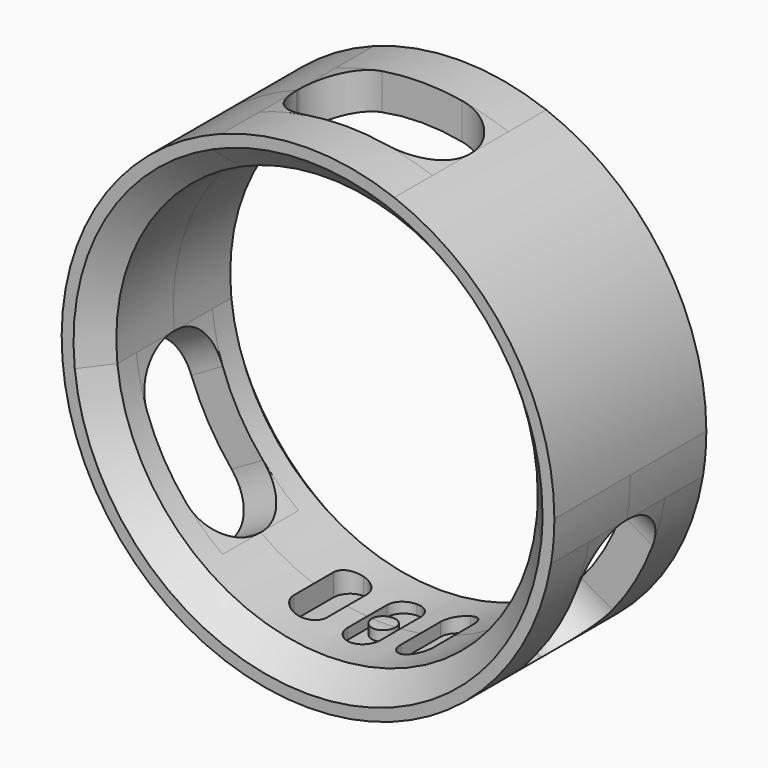
from build123d import *

# Parameters (mm, degrees)
F1_DEPTH      = 4
F1_DEPTH_BACK = 4
F2_SIZE       = 1
F4_DEPTH      = 2
F4_DEPTH_BACK = 2
F5_T4_DEPTH   = 11.3208024162
F5_S5_R       = 8.875
F5_T6_DEPTH   = 8
F5_S7_R       = 10.375
F5_T8_DEPTH   = 8
F5_T12_DEPTH  = 11.3208024162
F5_S13_R      = 10.375
F5_T14_DEPTH  = 8
F5_S15_R      = 8.875
F5_T16_DEPTH  = 8
F5_T20_DEPTH  = 11.3208024162
F5_S21_R      = 8.875
F5_T22_DEPTH  = 8
F5_S23_R      = 10.375
F5_T24_DEPTH  = 8
F5_T28_DEPTH  = 11.3208024162
F5_S29_R      = 8.875
F5_T30_DEPTH  = 8
F5_S31_R      = 10.375
F5_T32_DEPTH  = 8
F5_T36_DEPTH  = 11.3208024162
F5_S37_R      = 8.875
F5_T38_DEPTH  = 8
F5_S39_R      = 10.375
F5_T40_DEPTH  = 8
F5_T44_DEPTH  = 11.3208024162
F5_S45_R      = 8.875
F5_T46_DEPTH  = 8
F5_S47_R      = 10.375
F5_T48_DEPTH  = 8
F5_T52_DEPTH  = 11.3208024162
F5_S53_R      = 8.875
F5_T54_DEPTH  = 8
F5_S55_R      = 10.375
F5_T56_DEPTH  = 8
F5_T60_DEPTH  = 11.3208024162
F5_S61_R      = 8.875
F5_T62_DEPTH  = 8
F5_S63_R      = 10.375
F5_T64_DEPTH  = 8
F5_T68_DEPTH  = 11.3208024162
F5_S69_R      = 8.875
F5_T70_DEPTH  = 7
F5_S71_R      = 10.375
F5_T72_DEPTH  = 7
F5_T76_DEPTH  = 11.3208024162
F5_S77_R      = 8.875
F5_T78_DEPTH  = 7
F5_S79_R      = 10.375
F5_T80_DEPTH  = 7
F5_T84_DEPTH  = 11.3208024162
F5_S85_R      = 8.875
F5_T86_DEPTH  = 7
F5_S87_R      = 10.375
F5_T88_DEPTH  = 7
F5_T92_DEPTH  = 11.3208024162
F5_S93_R      = 8.875
F5_T94_DEPTH  = 7
F5_S95_R      = 10.375
F5_T96_DEPTH  = 7
F6_R          = 0.5
F7_DEPTH      = 9.3


# Not quite as in the source:
# - a fillet or chamfer that OpenCascade refuses, or shapes differently, is made with other operations: its cross-section is extruded or revolved along the edge and cut away or added


with BuildPart() as f1:
    # F0 (on Front) → F1 (new body, two sides)
    with BuildSketch(Plane.XZ) as f1_sk:
        with BuildLine():
            ThreePointArc((-3.6332620451, 8.0972237163), (0, 8.875), (3.6332620451, 8.0972237163))
            Line((3.6332620451, 8.0972237163), (3.6332620451, 9.7180261325))
            ThreePointArc((3.6332620451, 9.7180261325), (0, 10.375), (-3.6332620451, 9.7180261325))
            Line((-3.6332620451, 9.7180261325), (-3.6332620451, 8.0972237163))
        make_face()
        with BuildLine():
            ThreePointArc((-8.829032461, -0.9021146285), (-7.6859754586, 4.4375), (-3.6332620451, 8.0972237163))
            Line((-3.6332620451, 8.0972237163), (-3.6332620451, 9.7180261325))
            ThreePointArc((-3.6332620451, 9.7180261325), (-8.9850135643, 5.1875), (-10.2326885279, -1.7125158366))
            Line((-10.2326885279, -1.7125158366), (-8.829032461, -0.9021146285))
        make_face()
        with BuildLine():
            ThreePointArc((-5.1957704159, -7.1951090878), (-7.6859754586, -4.4375), (-8.829032461, -0.9021146285))
            Line((-8.829032461, -0.9021146285), (-10.2326885279, -1.7125158366))
            ThreePointArc((-10.2326885279, -1.7125158366), (-8.9850135643, -5.1875), (-6.5994264829, -8.0055102959))
            Line((-6.5994264829, -8.0055102959), (-5.1957704159, -7.1951090878))
        make_face()
        with BuildLine():
            Line((6.5994264829, -8.0055102959), (5.1957704159, -7.1951090878))
            ThreePointArc((5.1957704159, -7.1951090878), (0, -8.875), (-5.1957704159, -7.1951090878))
            Line((-5.1957704159, -7.1951090878), (-6.5994264829, -8.0055102959))
            ThreePointArc((-6.5994264829, -8.0055102959), (0, -10.375), (6.5994264829, -8.0055102959))
        make_face()
        with BuildLine():
            Line((10.2326885279, -1.7125158366), (8.829032461, -0.9021146285))
            ThreePointArc((8.829032461, -0.9021146285), (7.6859754586, -4.4375), (5.1957704159, -7.1951090878))
            Line((5.1957704159, -7.1951090878), (6.5994264829, -8.0055102959))
            ThreePointArc((6.5994264829, -8.0055102959), (8.9850135643, -5.1875), (10.2326885279, -1.7125158366))
        make_face()
        with BuildLine():
            ThreePointArc((3.6332620451, 8.0972237163), (7.450195489, 4.8228842175), (8.875, 0))
            ThreePointArc((8.875, 0), (8.8635006654, -0.4516425073), (8.829032461, -0.9021146285))
            Line((8.829032461, -0.9021146285), (10.2326885279, -1.7125158366))
            ThreePointArc((10.2326885279, -1.7125158366), (10.3393609202, -0.8592093816), (10.375, 0))
            ThreePointArc((10.375, 0), (8.524544525, 5.9137776118), (3.6332620451, 9.7180261325))
            Line((3.6332620451, 9.7180261325), (3.6332620451, 8.0972237163))
        make_face()
        with BuildLine():
            ThreePointArc((-5.1957704159, -7.1951090878), (-7.6859754586, -4.4375), (-8.829032461, -0.9021146285))
            Line((-8.829032461, -0.9021146285), (-10.2326885279, -1.7125158366))
            ThreePointArc((-10.2326885279, -1.7125158366), (-8.9850135643, -5.1875), (-6.5994264829, -8.0055102959))
            Line((-6.5994264829, -8.0055102959), (-5.1957704159, -7.1951090878))
        make_face()
        with BuildLine():
            ThreePointArc((3.6332620451, 8.0972237163), (7.450195489, 4.8228842175), (8.875, 0))
            ThreePointArc((8.875, 0), (8.8635006654, -0.4516425073), (8.829032461, -0.9021146285))
            Line((8.829032461, -0.9021146285), (10.2326885279, -1.7125158366))
            ThreePointArc((10.2326885279, -1.7125158366), (10.3393609202, -0.8592093816), (10.375, 0))
            ThreePointArc((10.375, 0), (8.524544525, 5.9137776118), (3.6332620451, 9.7180261325))
            Line((3.6332620451, 9.7180261325), (3.6332620451, 8.0972237163))
        make_face()
        with BuildLine():
            ThreePointArc((-8.829032461, -0.9021146285), (-7.6859754586, 4.4375), (-3.6332620451, 8.0972237163))
            Line((-3.6332620451, 8.0972237163), (-3.6332620451, 9.7180261325))
            ThreePointArc((-3.6332620451, 9.7180261325), (-8.9850135643, 5.1875), (-10.2326885279, -1.7125158366))
            Line((-10.2326885279, -1.7125158366), (-8.829032461, -0.9021146285))
        make_face()
        with BuildLine():
            ThreePointArc((-5.1957704159, -7.1951090878), (-7.6859754586, -4.4375), (-8.829032461, -0.9021146285))
            Line((-8.829032461, -0.9021146285), (-10.2326885279, -1.7125158366))
            ThreePointArc((-10.2326885279, -1.7125158366), (-8.9850135643, -5.1875), (-6.5994264829, -8.0055102959))
            Line((-6.5994264829, -8.0055102959), (-5.1957704159, -7.1951090878))
        make_face()
    extrude(amount=F1_DEPTH)
    extrude(f1_sk.sketch, amount=-F1_DEPTH_BACK)

    # F2
    f2_edges = [f1.edges().sort_by_distance(p)[0] for p in [
        (-8.829032, -4, 0.902115),
        (-8.829032, 4, 0.902115),
    ]]
    chamfer(f2_edges, length=F2_SIZE)

    # F0 (on Front) → F4 (cut, two sides)
    with BuildSketch(Plane.XZ) as f4_sk:
        with BuildLine():
            ThreePointArc((-3.6332620451, 9.7180261325), (0, 10.375), (3.6332620451, 9.7180261325))
            Line((3.6332620451, 9.7180261325), (3.6332620451, 11.8753320796))
            Line((3.6332620451, 11.8753320796), (-3.6332620451, 11.8753320796))
            Line((-3.6332620451, 11.8753320796), (-3.6332620451, 9.7180261325))
        make_face()
        with BuildLine():
            ThreePointArc((-3.6332620451, 8.0972237163), (0, 8.875), (3.6332620451, 8.0972237163))
            Line((3.6332620451, 8.0972237163), (3.6332620451, 9.7180261325))
            ThreePointArc((3.6332620451, 9.7180261325), (0, 10.375), (-3.6332620451, 9.7180261325))
            Line((-3.6332620451, 9.7180261325), (-3.6332620451, 8.0972237163))
        make_face()
        with BuildLine():
            Line((3.6332620451, 6.6060326062), (3.6332620451, 8.0972237163))
            ThreePointArc((3.6332620451, 8.0972237163), (0, 8.875), (-3.6332620451, 8.0972237163))
            Line((-3.6332620451, 8.0972237163), (-3.6332620451, 6.6060326062))
            Line((-3.6332620451, 6.6060326062), (3.6332620451, 6.6060326062))
        make_face()
        with BuildLine():
            ThreePointArc((5.1957704159, -7.1951090878), (7.6859754586, -4.4375), (8.829032461, -0.9021146285))
            Line((8.829032461, -0.9021146285), (7.2665240901, 0))
            Line((7.2665240901, 0), (3.3491878185, -6.1289841281))
            Line((3.3491878185, -6.1289841281), (5.1957704159, -7.1951090878))
        make_face()
        with BuildLine():
            Line((10.2326885279, -1.7125158366), (8.829032461, -0.9021146285))
            ThreePointArc((8.829032461, -0.9021146285), (7.6859754586, -4.4375), (5.1957704159, -7.1951090878))
            Line((5.1957704159, -7.1951090878), (6.5994264829, -8.0055102959))
            ThreePointArc((6.5994264829, -8.0055102959), (8.9850135643, -5.1875), (10.2326885279, -1.7125158366))
        make_face()
        with BuildLine():
            Line((12.1009702818, -2.7911688102), (10.2326885279, -1.7125158366))
            ThreePointArc((10.2326885279, -1.7125158366), (8.9850135643, -5.1875), (6.5994264829, -8.0055102959))
            Line((6.5994264829, -8.0055102959), (8.4677082368, -9.0841632694))
            Line((8.4677082368, -9.0841632694), (12.1009702818, -2.7911688102))
        make_face()
        with BuildLine():
            Line((-6.8559292529, 0.2370570398), (-8.829032461, -0.9021146285))
            ThreePointArc((-8.829032461, -0.9021146285), (-7.6859754586, -4.4375), (-5.1957704159, -7.1951090878))
            Line((-5.1957704159, -7.1951090878), (-3.2841431884, -6.0914305934))
            Line((-3.2841431884, -6.0914305934), (-6.8559292529, 0.2370570398))
        make_face()
        with BuildLine():
            ThreePointArc((-6.5994264829, -8.0055102959), (-8.9850135643, -5.1875), (-10.2326885279, -1.7125158366))
            Line((-10.2326885279, -1.7125158366), (-12.1009702818, -2.7911688102))
            Line((-12.1009702818, -2.7911688102), (-8.4677082368, -9.0841632694))
            Line((-8.4677082368, -9.0841632694), (-6.5994264829, -8.0055102959))
        make_face()
        with BuildLine():
            ThreePointArc((-5.1957704159, -7.1951090878), (-7.6859754586, -4.4375), (-8.829032461, -0.9021146285))
            Line((-8.829032461, -0.9021146285), (-10.2326885279, -1.7125158366))
            ThreePointArc((-10.2326885279, -1.7125158366), (-8.9850135643, -5.1875), (-6.5994264829, -8.0055102959))
            Line((-6.5994264829, -8.0055102959), (-5.1957704159, -7.1951090878))
        make_face()
    extrude(amount=-F4_DEPTH, mode=Mode.SUBTRACT)
    extrude(f4_sk.sketch, amount=F4_DEPTH_BACK, mode=Mode.SUBTRACT)

    # F5: fillet of radius 1.94 on 12 edges, made by hand


with BuildPart() as f5_tool2:
    # F5_s3 → F5_t4 (new body)
    with BuildSketch(Plane(origin=(2.8121782301, 0, -1.6236118582), x_dir=(0, 1, 0), z_dir=(0.8660254038, 0, -0.5))):
        with BuildLine():
            ThreePointArc((0.06, -3.6332620451), (1.4317871555, -3.0650492006), (2, -1.6932620451))
            Line((2, -1.6932620451), (2, -3.6332620451))
            Line((2, -3.6332620451), (0.06, -3.6332620451))
        make_face()
    extrude(amount=F5_T4_DEPTH)

    # F5_s5 → F5_t6 (cut, symmetric)
    with BuildSketch(Plane.XZ.offset(-1)):
        Circle(F5_S5_R)
    extrude(amount=F5_T6_DEPTH, both=True, mode=Mode.SUBTRACT)

    # F5_s7 → F5_t8 (intersect, symmetric)
    with BuildSketch(Plane.XZ.offset(-1)):
        Circle(F5_S7_R)
    extrude(amount=F5_T8_DEPTH, both=True, mode=Mode.INTERSECT)


with BuildPart() as f1_1:
    add(f1.part)

    # F5_t1: union F5_tool2
    add(f5_tool2.part)


with BuildPart() as f5_tool10:
    # F5_s11 → F5_t12 (new body)
    with BuildSketch(Plane(origin=(12.6162807137, 0, -7.2840130663), x_dir=(0, 1, 0), z_dir=(-0.8660254038, 0, 0.5))):
        with BuildLine():
            ThreePointArc((0.06, -3.6332620451), (1.4317871555, -3.0650492006), (2, -1.6932620451))
            Line((2, -1.6932620451), (2, -3.6332620451))
            Line((2, -3.6332620451), (0.06, -3.6332620451))
        make_face()
    extrude(amount=F5_T12_DEPTH)

    # F5_s13 → F5_t14 (intersect, symmetric)
    with BuildSketch(Plane.XZ.offset(-1)):
        Circle(F5_S13_R)
    extrude(amount=F5_T14_DEPTH, both=True, mode=Mode.INTERSECT)

    # F5_s15 → F5_t16 (cut, symmetric)
    with BuildSketch(Plane.XZ.offset(-1)):
        Circle(F5_S15_R)
    extrude(amount=F5_T16_DEPTH, both=True, mode=Mode.SUBTRACT)


with BuildPart() as f1_2:
    add(f1_1.part)

    # F5_t9: union F5_tool10
    add(f5_tool10.part)


with BuildPart() as f5_tool18:
    # F5_s19 → F5_t20 (new body)
    with BuildSketch(Plane(origin=(12.6162807137, 0, -7.2840130663), x_dir=(0, 1, 0), z_dir=(-0.8660254038, 0, 0.5))):
        with BuildLine():
            ThreePointArc((-0.06, -3.6332620451), (-1.4317871555, -3.0650492006), (-2, -1.6932620451))
            Line((-2, -1.6932620451), (-2, -3.6332620451))
            Line((-2, -3.6332620451), (-0.06, -3.6332620451))
        make_face()
    extrude(amount=F5_T20_DEPTH)

    # F5_s21 → F5_t22 (cut, symmetric)
    with BuildSketch(Plane.XZ.offset(1)):
        Circle(F5_S21_R)
    extrude(amount=F5_T22_DEPTH, both=True, mode=Mode.SUBTRACT)

    # F5_s23 → F5_t24 (intersect, symmetric)
    with BuildSketch(Plane.XZ.offset(1)):
        Circle(F5_S23_R)
    extrude(amount=F5_T24_DEPTH, both=True, mode=Mode.INTERSECT)


with BuildPart() as f1_3:
    add(f1_2.part)

    # F5_t17: union F5_tool18
    add(f5_tool18.part)


with BuildPart() as f5_tool26:
    # F5_s27 → F5_t28 (new body)
    with BuildSketch(Plane(origin=(2.8121782301, 0, -1.6236118582), x_dir=(0, 1, 0), z_dir=(0.8660254038, 0, -0.5))):
        with BuildLine():
            ThreePointArc((-2, -1.6932620451), (-1.4317871555, -3.0650492006), (-0.06, -3.6332620451))
            Line((-0.06, -3.6332620451), (-2, -3.6332620451))
            Line((-2, -3.6332620451), (-2, -1.6932620451))
        make_face()
    extrude(amount=F5_T28_DEPTH)

    # F5_s29 → F5_t30 (cut, symmetric)
    with BuildSketch(Plane.XZ.offset(1)):
        Circle(F5_S29_R)
    extrude(amount=F5_T30_DEPTH, both=True, mode=Mode.SUBTRACT)

    # F5_s31 → F5_t32 (intersect, symmetric)
    with BuildSketch(Plane.XZ.offset(1)):
        Circle(F5_S31_R)
    extrude(amount=F5_T32_DEPTH, both=True, mode=Mode.INTERSECT)


with BuildPart() as f1_4:
    add(f1_3.part)

    # F5_t25: union F5_tool26
    add(f5_tool26.part)


with BuildPart() as f5_tool34:
    # F5_s35 → F5_t36 (new body)
    with BuildSketch(Plane(origin=(-12.6162807137, 0, -7.2840130663), x_dir=(0, 1, 0), z_dir=(0.8660254038, 0, 0.5))):
        with BuildLine():
            ThreePointArc((0.06, -3.6332620451), (1.4317871555, -3.0650492006), (2, -1.6932620451))
            Line((2, -1.6932620451), (2, -3.6332620451))
            Line((2, -3.6332620451), (0.06, -3.6332620451))
        make_face()
    extrude(amount=F5_T36_DEPTH)

    # F5_s37 → F5_t38 (cut, symmetric)
    with BuildSketch(Plane.XZ.offset(-1)):
        Circle(F5_S37_R)
    extrude(amount=F5_T38_DEPTH, both=True, mode=Mode.SUBTRACT)

    # F5_s39 → F5_t40 (intersect, symmetric)
    with BuildSketch(Plane.XZ.offset(-1)):
        Circle(F5_S39_R)
    extrude(amount=F5_T40_DEPTH, both=True, mode=Mode.INTERSECT)


with BuildPart() as f1_5:
    add(f1_4.part)

    # F5_t33: union F5_tool34
    add(f5_tool34.part)


with BuildPart() as f5_tool42:
    # F5_s43 → F5_t44 (new body)
    with BuildSketch(Plane(origin=(-2.8121782301, 0, -1.6236118582), x_dir=(0, 1, 0), z_dir=(-0.8660254038, 0, -0.5))):
        with BuildLine():
            ThreePointArc((0.06, -3.6332620451), (1.4317871555, -3.0650492006), (2, -1.6932620451))
            Line((2, -1.6932620451), (2, -3.6332620451))
            Line((2, -3.6332620451), (0.06, -3.6332620451))
        make_face()
    extrude(amount=F5_T44_DEPTH)

    # F5_s45 → F5_t46 (cut, symmetric)
    with BuildSketch(Plane.XZ.offset(-1)):
        Circle(F5_S45_R)
    extrude(amount=F5_T46_DEPTH, both=True, mode=Mode.SUBTRACT)

    # F5_s47 → F5_t48 (intersect, symmetric)
    with BuildSketch(Plane.XZ.offset(-1)):
        Circle(F5_S47_R)
    extrude(amount=F5_T48_DEPTH, both=True, mode=Mode.INTERSECT)


with BuildPart() as f1_6:
    add(f1_5.part)

    # F5_t41: union F5_tool42
    add(f5_tool42.part)


with BuildPart() as f5_tool50:
    # F5_s51 → F5_t52 (new body)
    with BuildSketch(Plane(origin=(-2.8121782301, 0, -1.6236118582), x_dir=(0, 1, 0), z_dir=(-0.8660254038, 0, -0.5))):
        with BuildLine():
            ThreePointArc((-2, -1.6932620451), (-1.4317871555, -3.0650492006), (-0.06, -3.6332620451))
            Line((-0.06, -3.6332620451), (-2, -3.6332620451))
            Line((-2, -3.6332620451), (-2, -1.6932620451))
        make_face()
    extrude(amount=F5_T52_DEPTH)

    # F5_s53 → F5_t54 (cut, symmetric)
    with BuildSketch(Plane.XZ.offset(1)):
        Circle(F5_S53_R)
    extrude(amount=F5_T54_DEPTH, both=True, mode=Mode.SUBTRACT)

    # F5_s55 → F5_t56 (intersect, symmetric)
    with BuildSketch(Plane.XZ.offset(1)):
        Circle(F5_S55_R)
    extrude(amount=F5_T56_DEPTH, both=True, mode=Mode.INTERSECT)


with BuildPart() as f1_7:
    add(f1_6.part)

    # F5_t49: union F5_tool50
    add(f5_tool50.part)


with BuildPart() as f5_tool58:
    # F5_s59 → F5_t60 (new body)
    with BuildSketch(Plane(origin=(-12.6162807137, 0, -7.2840130663), x_dir=(0, 1, 0), z_dir=(0.8660254038, 0, 0.5))):
        with BuildLine():
            ThreePointArc((-0.06, -3.6332620451), (-1.4317871555, -3.0650492006), (-2, -1.6932620451))
            Line((-2, -1.6932620451), (-2, -3.6332620451))
            Line((-2, -3.6332620451), (-0.06, -3.6332620451))
        make_face()
    extrude(amount=F5_T60_DEPTH)

    # F5_s61 → F5_t62 (cut, symmetric)
    with BuildSketch(Plane.XZ.offset(1)):
        Circle(F5_S61_R)
    extrude(amount=F5_T62_DEPTH, both=True, mode=Mode.SUBTRACT)

    # F5_s63 → F5_t64 (intersect, symmetric)
    with BuildSketch(Plane.XZ.offset(1)):
        Circle(F5_S63_R)
    extrude(amount=F5_T64_DEPTH, both=True, mode=Mode.INTERSECT)


with BuildPart() as f1_8:
    add(f1_7.part)

    # F5_t57: union F5_tool58
    add(f5_tool58.part)


with BuildPart() as f5_tool66:
    # F5_s67 → F5_t68 (new body)
    with BuildSketch(Plane.XY.offset(14.5680261325)):
        with BuildLine():
            ThreePointArc((-3.6332620451, 0.06), (-3.0650492006, 1.4317871555), (-1.6932620451, 2))
            Line((-1.6932620451, 2), (-3.6332620451, 2))
            Line((-3.6332620451, 2), (-3.6332620451, 0.06))
        make_face()
    extrude(amount=-F5_T68_DEPTH)

    # F5_s69 → F5_t70 (cut, symmetric)
    with BuildSketch(Plane.XZ.offset(-1)):
        Circle(F5_S69_R)
    extrude(amount=F5_T70_DEPTH, both=True, mode=Mode.SUBTRACT)

    # F5_s71 → F5_t72 (intersect, symmetric)
    with BuildSketch(Plane.XZ.offset(-1)):
        Circle(F5_S71_R)
    extrude(amount=F5_T72_DEPTH, both=True, mode=Mode.INTERSECT)


with BuildPart() as f1_9:
    add(f1_8.part)

    # F5_t65: union F5_tool66
    add(f5_tool66.part)


with BuildPart() as f5_tool74:
    # F5_s75 → F5_t76 (new body)
    with BuildSketch(Plane.XY.offset(3.2472237163)):
        with BuildLine():
            ThreePointArc((3.6332620451, 0.06), (3.0650492006, 1.4317871555), (1.6932620451, 2))
            Line((1.6932620451, 2), (3.6332620451, 2))
            Line((3.6332620451, 2), (3.6332620451, 0.06))
        make_face()
    extrude(amount=F5_T76_DEPTH)

    # F5_s77 → F5_t78 (cut, symmetric)
    with BuildSketch(Plane.XZ.offset(-1)):
        Circle(F5_S77_R)
    extrude(amount=F5_T78_DEPTH, both=True, mode=Mode.SUBTRACT)

    # F5_s79 → F5_t80 (intersect, symmetric)
    with BuildSketch(Plane.XZ.offset(-1)):
        Circle(F5_S79_R)
    extrude(amount=F5_T80_DEPTH, both=True, mode=Mode.INTERSECT)


with BuildPart() as f1_10:
    add(f1_9.part)

    # F5_t73: union F5_tool74
    add(f5_tool74.part)


with BuildPart() as f5_tool82:
    # F5_s83 → F5_t84 (new body)
    with BuildSketch(Plane.XY.offset(14.5680261325)):
        with BuildLine():
            ThreePointArc((-3.6332620451, -0.06), (-3.0650492006, -1.4317871555), (-1.6932620451, -2))
            Line((-1.6932620451, -2), (-3.6332620451, -2))
            Line((-3.6332620451, -2), (-3.6332620451, -0.06))
        make_face()
    extrude(amount=-F5_T84_DEPTH)

    # F5_s85 → F5_t86 (cut, symmetric)
    with BuildSketch(Plane.XZ.offset(1)):
        Circle(F5_S85_R)
    extrude(amount=F5_T86_DEPTH, both=True, mode=Mode.SUBTRACT)

    # F5_s87 → F5_t88 (intersect, symmetric)
    with BuildSketch(Plane.XZ.offset(1)):
        Circle(F5_S87_R)
    extrude(amount=F5_T88_DEPTH, both=True, mode=Mode.INTERSECT)


with BuildPart() as f1_11:
    add(f1_10.part)

    # F5_t81: union F5_tool82
    add(f5_tool82.part)


with BuildPart() as f5_tool90:
    # F5_s91 → F5_t92 (new body)
    with BuildSketch(Plane.XY.offset(3.2472237163)):
        with BuildLine():
            ThreePointArc((1.6932620451, -2), (3.0650492006, -1.4317871555), (3.6332620451, -0.06))
            Line((3.6332620451, -0.06), (3.6332620451, -2))
            Line((3.6332620451, -2), (1.6932620451, -2))
        make_face()
    extrude(amount=F5_T92_DEPTH)

    # F5_s93 → F5_t94 (cut, symmetric)
    with BuildSketch(Plane.XZ.offset(1)):
        Circle(F5_S93_R)
    extrude(amount=F5_T94_DEPTH, both=True, mode=Mode.SUBTRACT)

    # F5_s95 → F5_t96 (intersect, symmetric)
    with BuildSketch(Plane.XZ.offset(1)):
        Circle(F5_S95_R)
    extrude(amount=F5_T96_DEPTH, both=True, mode=Mode.INTERSECT)


with BuildPart() as f1_12:
    add(f1_11.part)

    # F5_t89: union F5_tool90
    add(f5_tool90.part)

    # F6 (on Top) → F7 (cut)
    with BuildSketch(Plane.XY):
        with BuildLine():
            ThreePointArc((2.247434882, 1.7424248565), (1.7524601351, 1.5373996033), (1.547434882, 1.0424248565))
            Line((1.547434882, 1.0424248565), (1.547434882, -1.0499998212))
            ThreePointArc((1.547434882, -1.0499998212), (1.7524601351, -1.544974568), (2.247434882, -1.7499998212))
            ThreePointArc((2.247434882, -1.7499998212), (2.7424096288, -1.544974568), (2.947434882, -1.0499998212))
            Line((2.947434882, -1.0499998212), (2.947434882, 1.0424248565))
            ThreePointArc((2.947434882, 1.0424248565), (2.7424096288, 1.5373996033), (2.247434882, 1.7424248565))
        make_face()
        with BuildLine():
            ThreePointArc((-0.005565118, 1.7424248565), (-0.5005398649, 1.5373996033), (-0.705565118, 1.0424248565))
            Line((-0.705565118, 1.0424248565), (-0.705565118, -1.0499998212))
            ThreePointArc((-0.705565118, -1.0499998212), (-0.5005398649, -1.544974568), (-0.005565118, -1.7499998212))
            ThreePointArc((-0.005565118, -1.7499998212), (0.4894096288, -1.544974568), (0.694434882, -1.0499998212))
            Line((0.694434882, -1.0499998212), (0.694434882, 1.0424248565))
            ThreePointArc((0.694434882, 1.0424248565), (0.4894096288, 1.5373996033), (-0.005565118, 1.7424248565))
        make_face()
        with Locations((-0.0075767998, -0.0085298282)):
            Circle(F6_R, mode=Mode.SUBTRACT)
        with BuildLine():
            ThreePointArc((-2.2590144072, 1.7424248565), (-2.753989154, 1.5373996033), (-2.9590144072, 1.0424248565))
            Line((-2.9590144072, 1.0424248565), (-2.9590144072, -1.0499998212))
            ThreePointArc((-2.9590144072, -1.0499998212), (-2.753989154, -1.544974568), (-2.2590144072, -1.7499998212))
            ThreePointArc((-2.2590144072, -1.7499998212), (-1.7640396603, -1.544974568), (-1.5590144072, -1.0499998212))
            Line((-1.5590144072, -1.0499998212), (-1.5590144072, 1.0424248565))
            ThreePointArc((-1.5590144072, 1.0424248565), (-1.7640396603, 1.5373996033), (-2.2590144072, 1.7424248565))
        make_face()
    extrude(amount=-F7_DEPTH, mode=Mode.SUBTRACT)


solid = f1_12.part
